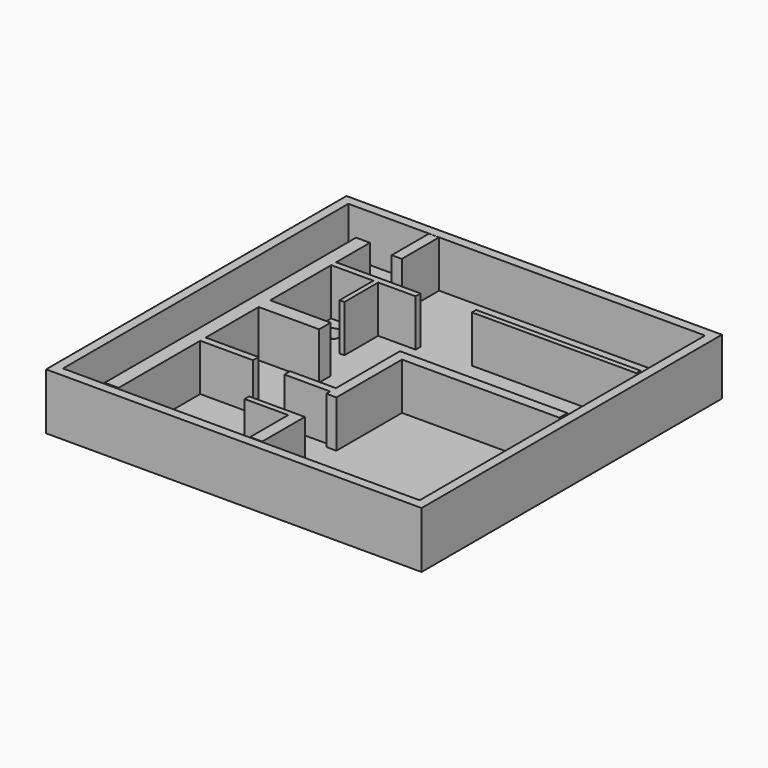
from build123d import *

# Parameters (mm, degrees)
F0_W      = 50.8
F0_H      = 50.8
F1_DEPTH  = 7.62
F2_T      = -1.27
F4_DEPTH  = 25.4
F5_DEPTH  = 6.35
F6_DEPTH  = 25.4
F8_DEPTH  = 6.35
F7_W      = 7.134902291
F7_H      = 0.9276261553
F7_W_2    = 0.6489050575
F7_H_2    = 5.7103633881
F7_R      = 1.27
F7_W_3    = 1.3627009466
F7_H_3    = 6.2943808734
F7_W_4    = 22.2574435174
F7_H_4    = 0.7137954235
F7_W_5    = 21.2840866297
F7_H_5    = 1.362701878
F7_W_6    = 6.2016416341
F7_H_6    = 0.982192345
F7_W_7    = 5.8931484818
F7_H_7    = 0.7639275864
F9_DEPTH  = 6.35
F10_DEPTH = 25.4
F11_DEPTH = 25.4


# Not quite as in the source:
# - a feature names something its author has since deleted; it is built from what else it names


with BuildPart() as f1:
    # F0 (on Top) → F1 (new body)
    with BuildSketch(Plane.XY):
        with Locations((25.4, 25.4)):
            Rectangle(F0_W, F0_H)
    extrude(amount=F1_DEPTH)

    # F2
    f2_openings = [f1.faces().sort_by_distance(p)[0] for p in [
        (25.4, 25.4, 7.62),
    ]]
    offset(amount=F2_T, openings=f2_openings)

    # F3 (on face) → F4 (cut)
    with BuildSketch(Plane.XY.offset(1.27)):
        with BuildLine():
            ThreePointArc((5.08, 3.81), (3.81, 5.08), (2.54, 3.81))
            Line((2.54, 3.81), (3.81, 3.81))
            Line((3.81, 3.81), (3.81, 2.54))
            ThreePointArc((3.81, 2.54), (4.7080256121, 2.9119743879), (5.08, 3.81))
        make_face()
        with BuildLine():
            Line((3.81, 3.81), (2.54, 3.81))
            ThreePointArc((2.54, 3.81), (2.9119743879, 2.9119743879), (3.81, 2.54))
            Line((3.81, 2.54), (3.81, 3.81))
        make_face()
    extrude(amount=-F4_DEPTH, mode=Mode.SUBTRACT)

    # F3 (on face) → F5 (cut)
    with BuildSketch(Plane.XY.offset(1.27)):
        with BuildLine():
            Line((1.27, 49.53), (1.27, 3.81))
            Line((1.27, 3.81), (2.54, 3.81))
            ThreePointArc((2.54, 3.81), (3.81, 5.08), (5.08, 3.81))
            ThreePointArc((5.08, 3.81), (4.7080256121, 2.9119743879), (3.81, 2.54))
            Line((3.81, 2.54), (3.81, 1.27))
            Line((3.81, 1.27), (49.53, 1.27))
            Line((49.53, 1.27), (49.53, 49.53))
            Line((49.53, 49.53), (1.27, 49.53))
        make_face()
    extrude(amount=F5_DEPTH, mode=Mode.SUBTRACT)

    # F3 (on face) → F6 (cut)
    with BuildSketch(Plane.XY.offset(1.27)):
        with BuildLine():
            ThreePointArc((5.08, 3.81), (3.81, 5.08), (2.54, 3.81))
            Line((2.54, 3.81), (3.81, 3.81))
            Line((3.81, 3.81), (3.81, 2.54))
            ThreePointArc((3.81, 2.54), (4.7080256121, 2.9119743879), (5.08, 3.81))
        make_face()
        with BuildLine():
            Line((3.81, 3.81), (2.54, 3.81))
            ThreePointArc((2.54, 3.81), (2.9119743879, 2.9119743879), (3.81, 2.54))
            Line((3.81, 2.54), (3.81, 3.81))
        make_face()
    extrude(amount=-F6_DEPTH, mode=Mode.SUBTRACT)

    # F7 (on face) → F8 (join)
    with BuildSketch(Plane.XY.offset(1.27)):
        Polygon((6.7439782433, 1.4878462534), (8.625802584, 1.4878462534), (8.625802584, 15.2857145295), (8.625802584, 16.2133406848), (8.625802584, 25.1728836447), (8.625802584, 27.1195974201), (8.625802584, 37.4371893704), (8.625802584, 38.2807664573), (8.625802584, 43.9911298454), (6.7439782433, 43.9911298454), align=None)
    extrude(amount=F8_DEPTH)

    # F7 (on face) → F9 (join)
    with BuildSketch(Plane.XY.offset(1.27)):
        Polygon((6.7439782433, 1.4878462534), (8.625802584, 1.4878462534), (8.625802584, 15.2857145295), (8.625802584, 16.2133406848), (8.625802584, 25.1728836447), (8.625802584, 27.1195974201), (8.625802584, 37.4371893704), (8.625802584, 38.2807664573), (8.625802584, 43.9911298454), (6.7439782433, 43.9911298454), align=None)
        with Locations((12.1932537295, 15.7495276071)):
            Rectangle(F7_W, F7_H)
        Polygon((8.625802584, 27.1195974201), (8.625802584, 25.1728836447), (16.8020073324, 25.1728836447), (16.8020073324, 25.9515698999), (16.8020073324, 27.1195974201), align=None)
        Polygon((20.0465321541, 38.2807664573), (8.625802584, 38.2807664573), (8.625802584, 37.4371893704), (14.336167369, 37.4371893704), (14.9850724265, 37.4371893704), (20.0465321541, 37.4371893704), align=None)
        with Locations((14.6606198978, 34.5820076764)):
            Rectangle(F7_W_2, F7_H_2)
        with Locations((10.7671897858, 34.7117893398)):
            Circle(F7_R)
        with Locations((3.3047813922, 9.144927375)):
            Circle(F7_R)
        with Locations((12.8761311062, 46.3596340269)):
            Rectangle(F7_W_3, F7_H_3)
        with Locations((38.118539378, 38.6376641691)):
            Rectangle(F7_W_4, F7_H_4)
        Polygon((27.963174507, 26.6004744917), (26.6004744917, 26.6004744917), (26.6004744917, 15.7768111676), (26.6004744917, 14.7946188226), (26.6004744917, 14.1414962709), (27.963174507, 14.1414962709), (27.963174507, 25.2377726138), align=None)
        with Locations((38.6052178219, 25.9191235527)):
            Rectangle(F7_W_5, F7_H_5)
        with Locations((23.4996536747, 15.2857149951)):
            Rectangle(F7_W_6, F7_H_6)
        with Locations((43.7315702438, 23.4208386391)):
            Circle(F7_R)
        Polygon((28.1472336501, 8.5740732029), (26.510246098, 8.5740732029), (26.510246098, 7.8101456165), (26.510246098, 1.3713347726), (28.1472336501, 1.3713347726), align=None)
        with Locations((23.5636718571, 8.1921094097)):
            Rectangle(F7_W_7, F7_H_7)
    extrude(amount=F9_DEPTH)

    # F10 (cut): faces of the model
    f10_faces = [f1.faces().sort_by_distance(p)[0] for p in [
        (10.7671897858, 34.7117893398, 7.62),
        (3.3047813922, 9.144927375, 7.62),
    ]]
    extrude(f10_faces, amount=-F10_DEPTH, mode=Mode.SUBTRACT)

    # F11 (cut): a face of the model
    f11_faces = [f1.faces().sort_by_distance(p)[0] for p in [
        (43.7315702438, 23.4208386391, 7.62),
    ]]
    extrude(f11_faces, amount=-F11_DEPTH, mode=Mode.SUBTRACT)


solid = f1.part
